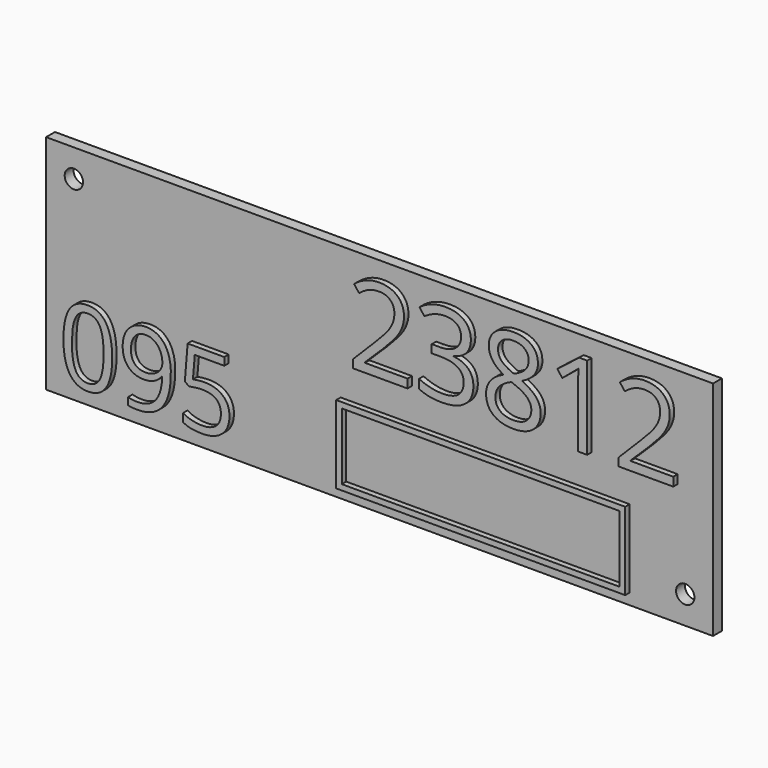
from build123d import *

# Parameters (mm, degrees)
F0_W         = 120
F0_H         = 40
F1_DEPTH     = 2
F3_D         = 3.3
F4_TEXT_SIZE = 20.9070615778
F5_DEPTH     = 1
F6_TEXT_SIZE = 18.5776487663
F7_DEPTH     = 1
F8_W         = 52
F8_H         = 14
F8_W_2       = 49.99999962
F8_H_2       = 11.99999962
F9_DEPTH     = 1


# Not quite as in the source:
# - Text() gives the source's letters only with a copy of the font that has no kerning and outlines rounded to 1/6400 em; it was checked with that copy


with BuildPart() as f1:
    # F0 (on Front) → F1 (new body)
    with BuildSketch(Plane.XZ):
        Rectangle(F0_W, F0_H)
    extrude(amount=F1_DEPTH)

    # F3 (through all)
    with Locations(Plane.XZ.offset(2)):
        with Locations((-55, 15), (55, -15)):
            Hole(F3_D / 2)

    # F4 (on face) → F5 (join)
    with BuildSketch(Plane.XZ.offset(2)):
        with Locations((-5, 2)):
            Text('23812', F4_TEXT_SIZE, font='Open Sans', text_align=(TextAlign.LEFT, TextAlign.BOTTOM))
    extrude(amount=F5_DEPTH)

    # F6 (on face) → F7 (join)
    with BuildSketch(Plane.XZ.offset(2)):
        with Locations((-57, -17)):
            Text('095', F6_TEXT_SIZE, font='Open Sans', text_align=(TextAlign.LEFT, TextAlign.BOTTOM))
    extrude(amount=F7_DEPTH)

    # F8 (on face) → F9 (join)
    with BuildSketch(Plane.XZ.offset(2)):
        with Locations((19, -11)):
            Rectangle(F8_W, F8_H)
        with Locations((19, -11)):
            Rectangle(F8_W_2, F8_H_2, mode=Mode.SUBTRACT)
    extrude(amount=F9_DEPTH)


solid = f1.part
